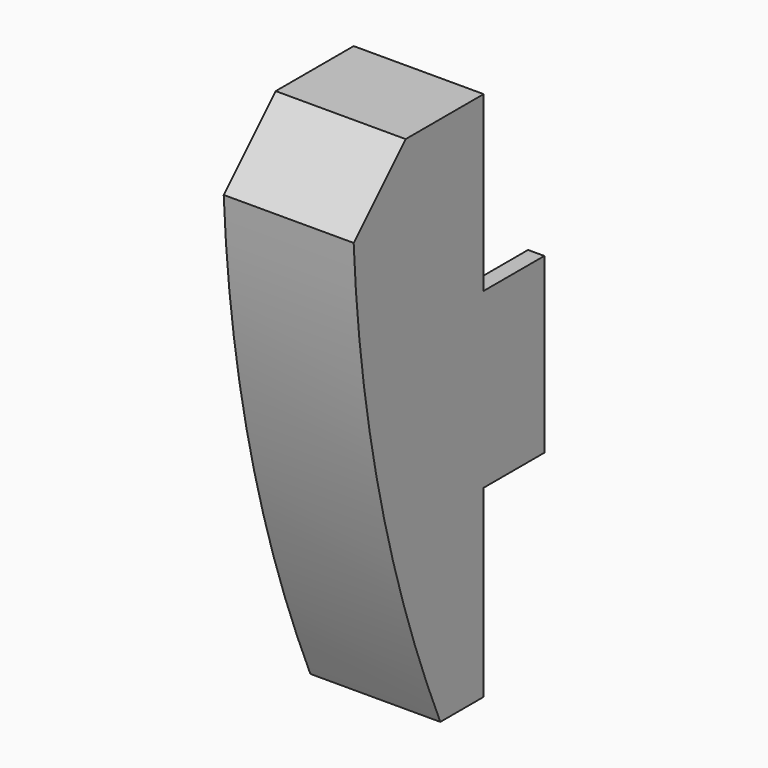
from build123d import *

# Parameters (mm, degrees)
F1_DEPTH      = 7.62
F0_W          = 3.81
F0_H          = 40.64
F2_DEPTH      = 17.78
F2_DEPTH_BACK = 7.62
F4_DEPTH      = 30.48
F6_DEPTH      = 50.8


# Not quite as in the source:
# - a feature names something its author has since deleted; it is built from what else it names


with BuildPart() as f1:
    # F0 (on Front) → F1 (new body)
    with BuildSketch(Plane.XZ):
        Polygon((-25.2661056346, 42.3477623217), (-55.7461056346, 42.3477623217), (-55.7461056346, 24.5677623217), (-51.9361056346, 24.5677623217), (-51.9361056346, -16.0722376783), (-55.7461056346, -16.0722376783), (-55.7461056346, -33.8522376783), (-25.2661056346, -33.8522376783), (-25.2661056346, -16.0722376783), (-29.0761056346, -16.0722376783), (-29.0761056346, 24.5677623217), (-25.2661056346, 24.5677623217), align=None)
    extrude(amount=F1_DEPTH)

    # F0 (on Front) → F2 (join, two sides)
    with BuildSketch(Plane.XZ) as f2_sk:
        with Locations((-53.8411056346, 4.2477623217)):
            Rectangle(F0_W, F0_H)
        with Locations((-27.1711056346, 4.2477623217)):
            Rectangle(F0_W, F0_H)
    extrude(amount=-F2_DEPTH)
    extrude(f2_sk.sketch, amount=F2_DEPTH_BACK)

    # F3 (on face) → F4 (join)
    with BuildSketch(Plane.YZ.offset(-25.2661056346)):
        with BuildLine():
            Line((-7.62, 42.3477623217), (0, 42.3477623217))
            Line((0, 42.3477623217), (0, 67.7477623217))
            Line((0, 67.7477623217), (-20.32, 67.7477623217))
            Line((-20.32, 67.7477623217), (-38.1, 49.9677623217))
            ThreePointArc((-38.1, 49.9677623217), (-30.341501455, -5.7914240632), (-12.7, -59.2522376783))
            Line((-12.7, -59.2522376783), (0, -59.2522376783))
            Line((0, -59.2522376783), (0, -33.8522376783))
            Line((0, -33.8522376783), (-7.62, -33.8522376783))
            Line((-7.62, -33.8522376783), (-7.62, 42.3477623217))
        make_face()
    extrude(amount=-F4_DEPTH)

    # F5 (on face) → F6 (cut)
    with BuildSketch(Plane.YZ.offset(-25.2661056346)):
        Polygon((0, 65.2077623217), (0, 67.7477623217), (-20.32, 67.7477623217), (-22.86, 65.2077623217), align=None)
    extrude(amount=-F6_DEPTH, mode=Mode.SUBTRACT)


solid = f1.part
